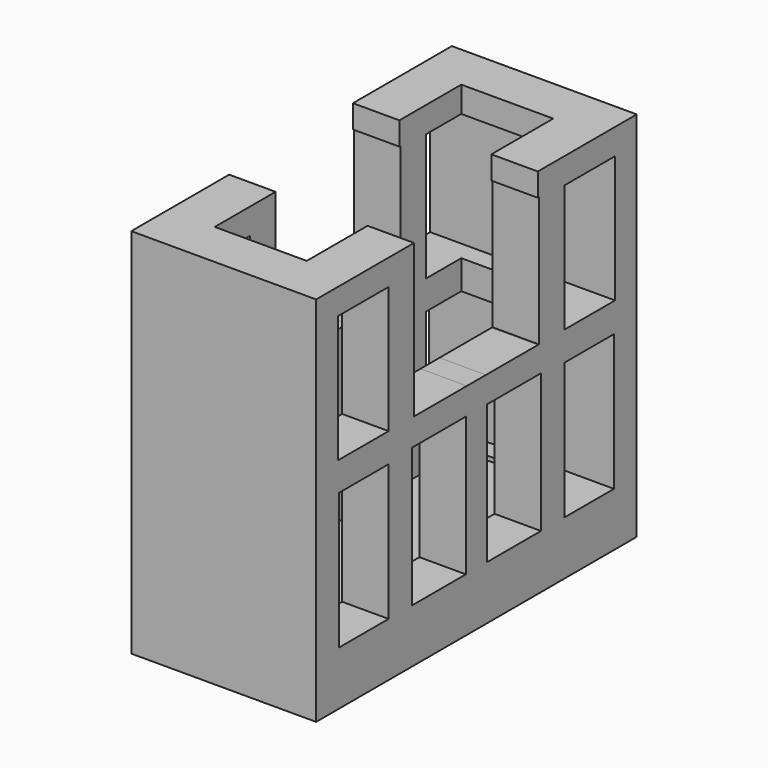
from build123d import *

# Parameters (mm, degrees)
F2_DEPTH = 60
F3_DEPTH = 52
F4_W     = 10.2412812412
F4_H     = 20.4825601541
F4_W_2   = 10.6680002064
F4_H_2   = 20.9092802834
F4_W_3   = 10.0279208273
F4_H_3   = 21.9760797918
F4_W_4   = 10.8813615516
F4_H_4   = 22.402798757
F5_DEPTH = 29.8242783788
F6_W     = 10.4546393268
F6_H     = 20.9092812147
F7_DEPTH = 29.8242783788


# Not quite as in the source:
# - ends of sketch curves that miss each other by under 0.0002 mm in the source are joined


with BuildPart() as f2:
    # F0 (on Top) → F2 (new body)
    with BuildSketch(Plane.XY):
        Polygon((-14.9116391894, 32.3240421712), (-14.9116391894, 24.8527319824), (-14.9116391894, -24.8527319824), (-14.9116391894, -32.3240421712), (14.9116391894, -32.3240421712), (14.9116391894, -24.8527319824), (14.9116391894, 24.8527319824), (14.9116391894, 32.3240421712), align=None)
        Polygon((-7.4186391894, 24.8527319824), (-0.0743608106, 24.8527319824), (0.0743608106, 24.8527319824), (7.4186391894, 24.8527319824), (7.4186391894, 0), (7.4186391894, -24.8527319824), (-7.4186391894, -24.8527319824), (-7.4186391894, 0), align=None, mode=Mode.SUBTRACT)
        Polygon((0.0743608106, 24.8527319824), (-0.0743608106, 24.8527319824), (-7.4186391894, 24.8527319824), (-7.4186391894, 0), (-7.4186391894, -24.8527319824), (7.4186391894, -24.8527319824), (7.4186391894, 0), (7.4186391894, 24.8527319824), align=None)
    extrude(amount=-F2_DEPTH)

    # F1 (on face) → F3 (cut)
    with BuildSketch(Plane.XY):
        Polygon((7.4186391894, 24.8527319824), (0.0743608106, 24.8527319824), (-0.0743608106, 24.8527319824), (-7.4186391894, 24.8527319824), (-7.4186391894, 0), (-7.4186391894, -24.8527319824), (7.4186391894, -24.8527319824), (7.4186391894, 0), align=None)
    extrude(amount=-F3_DEPTH, mode=Mode.SUBTRACT)

    # F4 (on face) → F5 (cut, through all)
    with BuildSketch(Plane.YZ.offset(14.9116391894)):
        with Locations((-22.8295195848, -14.401800232)):
            Rectangle(F4_W, F4_H)
        with Locations((-7.2542401031, -14.1884401673)):
            Rectangle(F4_W_2, F4_H_2)
        with Locations((7.2542401031, -14.1884401673)):
            Rectangle(F4_W_2, F4_H_2)
        with Locations((22.8295195848, -14.401800232)):
            Rectangle(F4_W, F4_H)
        with Locations((22.7228393778, -40.3250399977)):
            Rectangle(F4_W_3, F4_H_3)
        with Locations((7.5742793269, -40.1116805151)):
            Rectangle(F4_W_4, F4_H_4)
        with Locations((-7.5742793269, -40.1116805151)):
            Rectangle(F4_W_4, F4_H_4)
        with Locations((-22.7228393778, -40.3250399977)):
            Rectangle(F4_W_3, F4_H_3)
    extrude(amount=-F5_DEPTH, mode=Mode.SUBTRACT)

    # F6 (on face) → F7 (cut, through all)
    with BuildSketch(Plane(origin=(-14.9116391894, 0, 0), x_dir=(0, -1, 0), z_dir=(-1, 0, 0))):
        Polygon((12.5882383436, 0), (-12.3748793267, 0), (-12.3748793267, -3.7338000257), (-1.9202399999, -3.7338000257), (-1.9202399999, -24.643080309), (1.9202399999, -24.6430812404), (1.9202399999, -3.7338000257), (12.5882402062, -3.7338000257), align=None)
        with Locations((-7.1475596633, -14.188440633)):
            Rectangle(F6_W, F6_H)
        Polygon((12.5882383436, -24.6430812404), (12.5882383436, -3.7338000257), (1.9202399999, -3.7338000257), (1.9202399999, -24.643080309), align=None)
    extrude(amount=-F7_DEPTH, mode=Mode.SUBTRACT)


solid = f2.part
